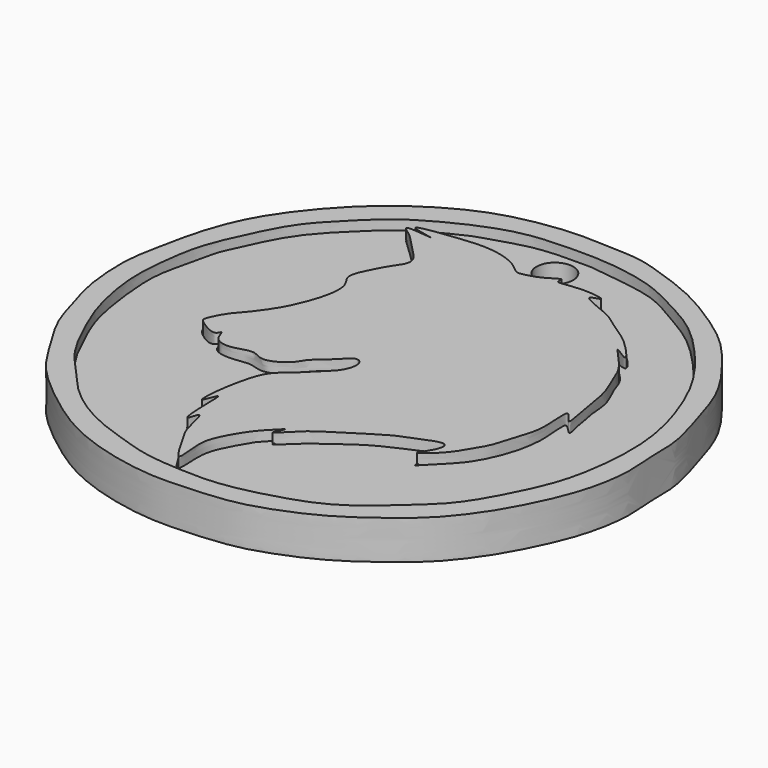
from build123d import *

# Parameters (mm, degrees)
F4_DEPTH  = 4
F5_DEPTH  = 4
F2_R      = 1.8820545133
F6_DEPTH  = 3
F8_R      = 1.5846941297
F9_DEPTH  = 4
F10_DEPTH = 4


# Not quite as in the source:
# - the program builds the solid bodies; features that only make, move or delete a surface that nothing else refers to are left out


with BuildPart() as f4:
    # F0 (on Top) → F4 (new body)
    with BuildSketch(Plane.XY):
        with BuildLine():
            add(Edge.make_bspline(
                [(18.5562651604, 42.7909307182), (18.4215312664, 42.3851537945), (17.7158013258, 41.5037860124), (17.0959159307, 40.2248370679), (15.9498157243, 38.0243570023), (17.2506828561, 36.8609286786), (17.1295075869, 34.7040352941), (16.5126368457, 32.7369497504), (15.5560201527, 30.4549243196), (13.7575389714, 28.0153669618), (12.799175522, 27.1380779485), (11.7664702912, 25.1092464404), (12.0644178962, 24.6377745601), (14.2068836882, 23.2585077591), (14.4431797453, 24.5650291399), (14.7668726498, 22.7324394766), (16.7197447937, 22.4212784818), (18.6585147185, 23.3755519954), (19.8677432958, 22.1399886507), (22.2820258178, 23.475839523), (22.6759274542, 24.7446848849), (24.3394334554, 25.8674199186), (25.7163404014, 27.673856323), (26.7246403482, 26.6948668964), (26.1077707678, 24.853744914), (24.8349029838, 23.8713129942), (23.5459555247, 22.3636054211), (21.6051700554, 21.0567176114), (20.8855115902, 18.1846513508), (20.4684690456, 15.8593397967), (20.4031366598, 13.1908179059), (21.3827274427, 16.5195865408), (21.1977723963, 12.5942008838), (21.5713420529, 10.0529993754), (22.0517066208, 12.8528846205), (22.6672650745, 9.0962128738), (23.5105387934, 7.9905387358), (25.7120553776, 3.8071318202), (25.020360857, 7.7221211031), (25.4013400752, 9.5027043321), (27.049373534, 12.3503159023), (28.2612591698, 13.4778262696), (29.2808044669, 14.5823030172), (27.8801976017, 12.2261155071), (30.3099720155, 14.9238371622), (31.5947274367, 15.7562814954), (34.4593332527, 17.5711478867), (36.4429250734, 18.8446399817), (37.9963600524, 19.3290924441), (40.8244094992, 20.6718959329), (40.7960751542, 19.0410089382), (39.0151197311, 16.7713540352), (41.725052143, 19.0850921358), (42.5271955302, 20.5907614593), (43.7358175787, 22.4157083215), (44.2251149078, 24.8498897974), (45.2233714127, 26.9757582349), (44.4540408444, 31.7310478503), (46.2913625604, 28.4192392382), (45.4338755154, 32.1192026142), (45.1113570416, 35.226951008), (43.9820222123, 37.3322163895), (43.4732705667, 39.3393485937), (39.9911596004, 42.6019596569), (43.5577244369, 39.9654020424), (40.5038196091, 43.4376664958), (38.3947815651, 44.5207456109), (36.9145549877, 45.9591536843), (32.6604656637, 47.2824882771), (35.5825197314, 47.7323829467), (31.9546510246, 48.2329346842), (29.7314391091, 47.5171719167), (30.2377357158, 48.7248556611), (28.7324648277, 47.5138023996), (27.0542248202, 47.1094932445), (26.3119347157, 46.9733193591), (25.2010011638, 48.2395026019), (22.1605808772, 49.0970593612), (19.0401320473, 48.7604989113), (13.4462899188, 48.0856491671), (19.148773227, 47.2032299486), (13.7332927421, 47.9583609124), (15.7575699724, 46.8145599642), (16.8043575059, 45.4306303515), (18.5829455142, 43.919181945), (18.6682894636, 43.1283133601), (18.5562651604, 42.7909307182)],
                knots=[0, 0, 0, 0, 0.0103611569, 0.0211009944, 0.033754164, 0.044100949, 0.0562398894, 0.0686091251, 0.0822990694, 0.0969469949, 0.1073320082, 0.1195065024, 0.1259227197, 0.138435722, 0.1444315201, 0.1535054216, 0.1650833387, 0.1771394308, 0.1872338073, 0.2003856482, 0.2101722739, 0.2224140673, 0.2344058097, 0.2422751457, 0.2536055817, 0.264581445, 0.2765484592, 0.2894335308, 0.3037607621, 0.3182385672, 0.3283063767, 0.3381433484, 0.3522284916, 0.3634704949, 0.3720936096, 0.3850882395, 0.3980805625, 0.4125499541, 0.4252446536, 0.4380290253, 0.4531596976, 0.4651328446, 0.4721278574, 0.4810934696, 0.4935980633, 0.5058858669, 0.5213799674, 0.5344683998, 0.5460530826, 0.5595476758, 0.5684008558, 0.5796093357, 0.5921302069, 0.604457496, 0.6168044353, 0.6299671409, 0.6443781962, 0.6592432859, 0.6691356229, 0.6818689832, 0.698352566, 0.7109611061, 0.7245719517, 0.7389139172, 0.7494654142, 0.7635793549, 0.7778764894, 0.7911499194, 0.8060608822, 0.8141792164, 0.8278014036, 0.8401293462, 0.845805421, 0.8557469209, 0.8676299668, 0.8744147147, 0.8848375473, 0.899566373, 0.9167400121, 0.9319443843, 0.9440842213, 0.9576621998, 0.9661241595, 0.9786232958, 0.9913852309, 1, 1, 1, 1], degree=3))
        make_face()
    extrude(amount=F4_DEPTH)


with BuildPart() as f5:
    # F1 (on Top) → F5 (new body)
    with BuildSketch(Plane.XY):
        with BuildLine():
            add(Edge.make_bspline(
                [(34.4799309969, 54.499745369), (35.6262734965, 54.1454744681), (38.6148886488, 53.1073992428), (41.747190705, 51.4886281676), (46.5271984131, 48.30305899), (48.7349391227, 45.5303297651), (50.3893973092, 43.5038502258), (52.4163505586, 40.3586870772), (53.5671900995, 36.2879620461), (54.9554152261, 32.1080573627), (54.7771465189, 28.7269471157), (55.2220669883, 25.5503672167), (54.3845303113, 20.4795987753), (52.0412754304, 15.5835601348), (50.4356791278, 12.8631726149), (48.292614741, 10.0423571222), (46.125559851, 8.1107725162), (43.0195109957, 5.7321159144), (39.874291258, 3.8178411097), (35.8374786296, 2.2318456408), (32.7975817845, 1.4745262164), (27.4004629786, 1.1457827562), (24.3278279133, 1.2669997026), (19.8586756582, 2.1396739435), (15.5315115107, 3.8373040418), (11.7877995558, 6.3951788076), (7.4582549601, 9.9582616609), (5.5244195076, 13.0876398049), (2.8066476892, 17.4264849603), (2.1625871244, 20.1634074923), (1.1675164824, 22.9541806386), (0.6881440402, 26.4162035447), (0.6607573929, 29.744948627), (1.2252376004, 32.4255381807), (2.0092644714, 36.5407169863), (3.6352216726, 41.0045497356), (6.6049876085, 45.2768074675), (10.2635155584, 49.1145557987), (14.1526146099, 51.8772366999), (19.0928448574, 54.4458976525), (25.804290261, 55.424495133), (28.9726980587, 55.1304435607), (32.2469035908, 55.1189682952), (33.6186751723, 54.7659117869), (34.4799309969, 54.499745369)],
                knots=[0, 0, 0, 0, 0.0243896001, 0.0474965162, 0.0758374539, 0.098220674, 0.1172300945, 0.1399534535, 0.1647467823, 0.1896995745, 0.211270068, 0.2323456767, 0.2593538122, 0.287125144, 0.3084500624, 0.3304002471, 0.3508601167, 0.3741632631, 0.3974001588, 0.42174148, 0.4433385661, 0.4705684117, 0.49189457, 0.5169099576, 0.5425849472, 0.5682050196, 0.5959759518, 0.6193269077, 0.6458779194, 0.665899734, 0.6860931079, 0.708497913, 0.7300572758, 0.7496925296, 0.7738661376, 0.7999201769, 0.8270930958, 0.8544276454, 0.8802282297, 0.908575656, 0.9392866471, 0.9608504911, 0.9816759082, 1, 1, 1, 1], degree=3))
        make_face()
        with BuildLine():
            add(Edge.make_bspline(
                [(20.3378461301, 51.9694536924), (19.1742040201, 51.5589848153), (16.7467459788, 50.4714875874), (13.1554017472, 48.4263577047), (10.7570419663, 46.1249510076), (7.6651545497, 43.0606317144), (6.0423672568, 40.0584684616), (4.5938121829, 36.9235718565), (3.543081208, 34.2387282175), (3.0290665941, 30.4357317654), (2.8151974269, 27.3697396453), (3.2468744753, 24.0794883971), (4.0048614958, 20.890418552), (5.7202121433, 17.0403948912), (7.4146900027, 13.7380673731), (9.7998009044, 11.3913492298), (11.3481492859, 9.4187665131), (13.4615640025, 7.5907219479), (16.4437076174, 5.8564429156), (19.6675884735, 4.792050307), (22.9975710995, 3.662491064), (26.7450478189, 3.4259616783), (30.8610364154, 3.2791620404), (36.6739212336, 4.7825332589), (40.7944648743, 6.4220223412), (45.0085013952, 10.1526996405), (47.8637606999, 12.7940087998), (50.0142009203, 16.704069632), (51.8438259294, 20.5413302587), (52.7808801285, 24.968806016), (53.0660590919, 30.7501211565), (51.7469460875, 35.9822399744), (49.615463109, 40.9166012264), (46.5817329215, 44.9333503398), (43.0085466455, 48.5663484826), (39.3748099722, 50.3891920662), (36.2883093918, 52.0924038667), (31.5309870375, 52.9926164731), (27.8522542002, 53.0367908812), (23.6510488502, 52.9267863037), (21.4320414638, 52.35542557), (20.3378461301, 51.9694536924)],
                knots=[0, 0, 0, 0, 0.0254094476, 0.0513741225, 0.0750118623, 0.1015873137, 0.1255620904, 0.1491587738, 0.1711410989, 0.1961193061, 0.218880845, 0.2419761496, 0.2653618033, 0.2917382127, 0.3167095418, 0.3399762576, 0.360233429, 0.381550882, 0.4053960625, 0.4291739932, 0.4531994553, 0.4778364378, 0.5041084793, 0.5353250691, 0.5628157382, 0.5928587943, 0.6184234564, 0.6452280828, 0.6716971041, 0.6989809519, 0.7297879583, 0.7597340465, 0.7893484345, 0.8182965762, 0.8472216219, 0.872859188, 0.8970336379, 0.9249739338, 0.9500533241, 0.9761070016, 1, 1, 1, 1], degree=3))
        make_face(mode=Mode.SUBTRACT)
    extrude(amount=F5_DEPTH)


with BuildPart() as f6:
    # F2 (on Top) → F6 (new body)
    with BuildSketch(Plane.XY):
        with BuildLine():
            add(Edge.make_bspline(
                [(5.9724645689, 40.0622151792), (5.4897215696, 39.1468696857), (4.4484015533, 37.2763130428), (3.8807857684, 33.8717669388), (2.8912729692, 30.4222986677), (3.0307767014, 27.2594263771), (3.4076838641, 24.1122830977), (4.0533332189, 20.7102083123), (5.6639694444, 17.2330893379), (7.3232557243, 13.6820080946), (9.6659735238, 11.5777426668), (11.3122586295, 9.3555552377), (13.578698674, 7.8367909149), (16.3640742068, 5.9159468873), (19.3455503336, 4.7955139976), (22.9612653874, 3.9230273268), (26.5015685348, 3.3170417249), (30.7949273613, 3.445949784), (36.8354130711, 4.6933121479), (40.912322393, 6.5494910163), (45.13201504, 10.1019636396), (47.793028087, 12.9215213904), (50.1604864739, 16.6435325725), (51.672356085, 20.4474309989), (52.8527392465, 24.4105543519), (53.1155807505, 30.7305744808), (51.5695536165, 35.6211075635), (49.7778626051, 40.7404590874), (46.5361436314, 44.7046135017), (43.0935242681, 48.2416634833), (39.2880770509, 50.3035440307), (36.4679404793, 52.0819500268), (31.5609731444, 52.7156842289), (27.8944813107, 53.2415795448), (23.4726280744, 52.8411743616), (20.5799504892, 51.8786164501), (16.5856723516, 50.7122026783), (13.0764708733, 48.1679800435), (10.7277216617, 46.3373632178), (7.4930291441, 43.0629376964), (6.4734051255, 41.0120656827), (5.9724645689, 40.0622151792)],
                knots=[0, 0, 0, 0, 0.0227841519, 0.0466988604, 0.0710552837, 0.0938261999, 0.1166773955, 0.1405333706, 0.1658708078, 0.1912946359, 0.2140047963, 0.2351238092, 0.256323601, 0.2798805099, 0.3029442569, 0.3276609909, 0.3518835762, 0.378652636, 0.4104308195, 0.4380411961, 0.4678236254, 0.4934223592, 0.5201779803, 0.5460532392, 0.572296509, 0.6043118418, 0.6337285785, 0.663399679, 0.6925022336, 0.7211525435, 0.7475890325, 0.7710875738, 0.7992278558, 0.8246253481, 0.8512056356, 0.8738381548, 0.8999834687, 0.9265448624, 0.9491074439, 0.9763569731, 1, 1, 1, 1], degree=3))
        make_face()
        with BuildLine():
            add(Edge.make_bspline(
                [(18.3281805366, 43.7832251191), (18.5845792486, 43.3876240235), (18.9147650049, 42.5426992126), (17.5549506598, 41.9674861095), (17.1548079959, 39.9504866207), (16.0838680334, 38.3325056903), (17.2044287518, 34.8835562858), (16.577827187, 32.5758220884), (15.1880480547, 30.3720998613), (13.8881620773, 27.8481028608), (12.333811938, 27.1250990792), (11.6177533691, 25.2007566358), (12.0158415824, 24.5020876227), (14.0529914521, 23.0770267776), (14.5429005942, 24.4961259463), (14.5111070009, 22.7334389414), (16.7656878153, 22.4234192994), (18.5601193435, 22.9449028943), (19.9297205235, 22.1091115796), (22.2805847106, 23.1735749389), (22.8089292905, 24.6741162525), (24.4095107441, 25.9480075789), (25.7673257518, 27.180818804), (26.9664108312, 26.7392707514), (25.8720682158, 24.9618337027), (24.8467802674, 23.6931720718), (23.4973694081, 22.3320297593), (21.6007290808, 21.2928067974), (20.7817250048, 18.0121996509), (20.488560769, 15.7681861662), (20.3581626069, 13.1483841947), (21.6074094082, 16.4218601118), (20.9093120798, 12.68183479), (21.5646138791, 10.0228726674), (22.1293538479, 12.8899594107), (22.6120525378, 9.1594605987), (23.4788873863, 7.7392719947), (25.6756927003, 3.6519658298), (25.1673606709, 7.6606984491), (25.6300736419, 9.5866014116), (27.0390779523, 12.0046142428), (27.9874188083, 13.6559341848), (29.4828420399, 14.4205531591), (27.9854735017, 12.1675225943), (30.2674684172, 14.5823657552), (31.7967031896, 15.6580738819), (34.3005277954, 17.5103678355), (36.4112207707, 18.5817485395), (38.2802940029, 19.3649677637), (40.5804906515, 20.4442809159), (40.9341532955, 19.1419144626), (38.9329199277, 16.2622525767), (41.6212639193, 19.088134865), (42.6971291613, 20.1889771637), (44.0526680389, 22.4385611029), (45.4195710943, 26.7555687241), (44.3802491658, 31.3127836996), (46.5199228426, 28.4507857395), (45.1499707505, 32.1572341067), (45.3941689935, 35.1613933518), (43.9073777822, 37.5566928824), (43.7206369429, 39.2908392258), (40.2482614366, 41.8828299847), (43.4140846389, 40.2933714561), (40.7073160013, 43.426448313), (38.3498316556, 44.5192168903), (36.9017918339, 45.8212475022), (32.9809751403, 47.0297422988), (35.5010798945, 47.7742399172), (32.2117382341, 48.3122748091), (30.4283364967, 48.1231387492), (30.063102547, 48.2529764636), (28.9009555949, 47.4429034848), (27.1356395243, 47.0718230527), (26.4449945422, 46.8911032234), (25.1934736758, 48.497670752), (22.48627191, 49.0370498887), (18.9333376393, 49.0855783912), (14.0609008283, 48.3772535849), (18.5905063036, 47.0695641355), (14.1589333133, 47.8591047175), (15.5725630031, 46.6651241434), (16.9673108062, 45.2833828644), (17.9906137466, 44.3040615576), (18.3281805366, 43.7832251191)],
                knots=[0, 0, 0, 0, 0.0093954215, 0.018800898, 0.0309600125, 0.0429538602, 0.0590206917, 0.0724200819, 0.0865990816, 0.1010829532, 0.1124375078, 0.1240634169, 0.1320368354, 0.1445948075, 0.1515412109, 0.160022142, 0.1724601058, 0.1844029258, 0.1949111293, 0.2080732563, 0.2189511175, 0.231476017, 0.2431229695, 0.2506069362, 0.2620050545, 0.2737377446, 0.2856034466, 0.2981448213, 0.3136683476, 0.3282389115, 0.3383635896, 0.3485806432, 0.3624879576, 0.3743483749, 0.3833714522, 0.3964504543, 0.4105435228, 0.4251352933, 0.4384154727, 0.4518148652, 0.4661692234, 0.4789221664, 0.4867484258, 0.4960549462, 0.5080958043, 0.5215889107, 0.5367132958, 0.550153618, 0.5631162207, 0.5757711535, 0.5841577371, 0.5967150885, 0.6098662297, 0.621906979, 0.6354487923, 0.6552075258, 0.6700991609, 0.679939948, 0.6933393382, 0.7097533517, 0.7235789744, 0.7361363307, 0.7503156232, 0.7597116965, 0.773658332, 0.7886764727, 0.8018526312, 0.8166437983, 0.8246960497, 0.8379321266, 0.850323686, 0.8550932095, 0.8651793531, 0.8771030741, 0.8838481882, 0.8953913169, 0.909588069, 0.9277498495, 0.9425136268, 0.9537902768, 0.9666364068, 0.974479127, 0.9876302721, 1, 1, 1, 1], degree=3))
        make_face(mode=Mode.SUBTRACT)
        with Locations((27.7375038713, 50.332210958)):
            Circle(F2_R, mode=Mode.SUBTRACT)
    extrude(amount=F6_DEPTH)

    # F8 (on face) → F9 (join)
    with BuildSketch(Plane.XY.offset(3)):
        with Locations((26.687450707, 51.1875003576)):
            Circle(F8_R)
    extrude(amount=F9_DEPTH)

    # F10 (cut): a face of the model
    f10_faces = [f6.faces().sort_by_distance(p)[0] for p in [
        (26.687450707, 51.1875003576, 7),
    ]]
    extrude(f10_faces, amount=-F10_DEPTH, mode=Mode.SUBTRACT)


solid = Compound([f4.part, f5.part, f6.part])
